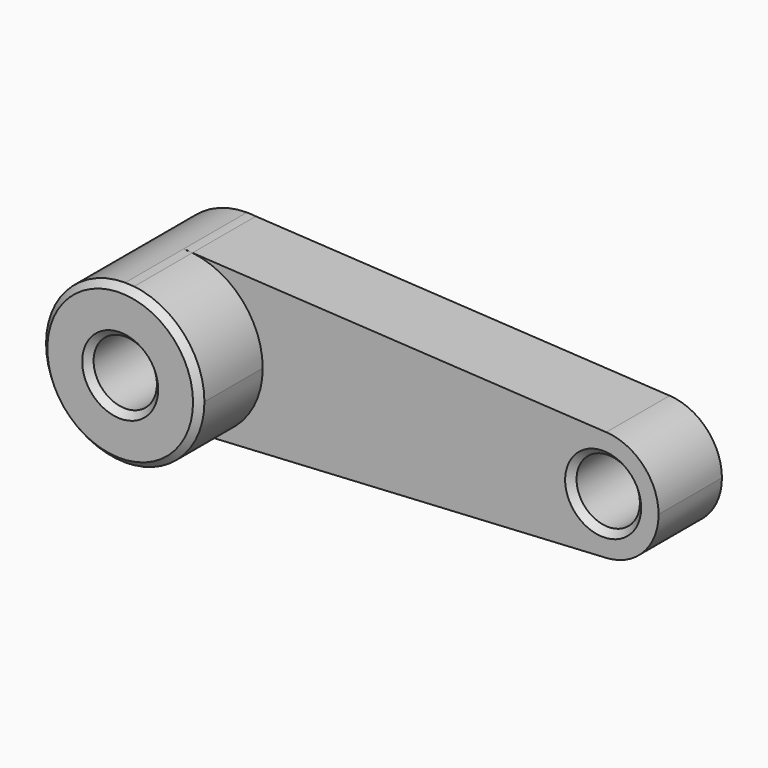
from build123d import *

# Parameters (mm, degrees)
F0_R        = 10
F1_DEPTH    = 25
F2_DEPTH    = 50
F3_T4_ANGLE = 203.6133668192
F3_T6_ANGLE = 179.9906971182


# Not quite as in the source:
# - a fillet or chamfer that OpenCascade refuses, or shapes differently, is made with other operations: its cross-section is extruded or revolved along the edge and cut away or added


with BuildPart() as f1:
    # F0 (on Front) → F1 (new body)
    with BuildSketch(Plane.XZ):
        with BuildLine():
            Line((2.8107571296, 24.8414903812), (0, 25))
            ThreePointArc((0, 25), (-25, 0), (0, -25))
            Line((0, -25), (2.8107571296, -24.8414903812))
            ThreePointArc((2.8107571296, -24.8414903812), (18.6449581421, -16.6542948179), (25, 0))
            ThreePointArc((25, 0), (18.6449581421, 16.6542948179), (2.8107571296, 24.8414903812))
        make_face()
        Circle(F0_R, mode=Mode.SUBTRACT)
        with BuildLine():
            ThreePointArc((2.8107571296, 24.8414903812), (1.4076115356, 24.9603411388), (0, 25))
            Line((0, 25), (2.8107571296, 24.8414903812))
        make_face()
        with BuildLine():
            Line((2.8107571296, -24.8414903812), (0, -25))
            ThreePointArc((0, -25), (1.4076115356, -24.9603411388), (2.8107571296, -24.8414903812))
        make_face()
        with BuildLine():
            Line((133.4853280749, 17.4722387972), (2.8107571296, 24.8414903812))
            ThreePointArc((2.8107571296, 24.8414903812), (18.6449581421, 16.6542948179), (25, 0))
            ThreePointArc((25, 0), (18.6449581421, -16.6542948179), (2.8107571296, -24.8414903812))
            Line((2.8107571296, -24.8414903812), (133.4853280749, -17.4722387972))
            ThreePointArc((133.4853280749, -17.4722387972), (115, 0), (133.4853280749, 17.4722387972))
        make_face()
        with BuildLine():
            ThreePointArc((150, 0), (145.2179644855, 12.0209558415), (133.4853280749, 17.4722387972))
            ThreePointArc((133.4853280749, 17.4722387972), (115, 0), (133.4853280749, -17.4722387972))
            ThreePointArc((133.4853280749, -17.4722387972), (145.2179644855, -12.0209558415), (150, 0))
        make_face()
        with Locations((132.5, 0)):
            Circle(F0_R, mode=Mode.SUBTRACT)
    extrude(amount=F1_DEPTH)

    # F0 (on Front) → F2 (join)
    with BuildSketch(Plane.XZ):
        with BuildLine():
            Line((2.8107571296, 24.8414903812), (0, 25))
            ThreePointArc((0, 25), (-25, 0), (0, -25))
            Line((0, -25), (2.8107571296, -24.8414903812))
            ThreePointArc((2.8107571296, -24.8414903812), (18.6449581421, -16.6542948179), (25, 0))
            ThreePointArc((25, 0), (18.6449581421, 16.6542948179), (2.8107571296, 24.8414903812))
        make_face()
        Circle(F0_R, mode=Mode.SUBTRACT)
    extrude(amount=F2_DEPTH)

    # F3: chamfer of 2 on 4 edges, made by hand

    # F3_s1 → F3_t2 (revolve, cut)
    with BuildSketch(Plane.XY):
        Polygon((12, -50), (10, -48), (10, -50), align=None)
    revolve(axis=Axis((0, -50, 0), (0, -1, 0)), mode=Mode.SUBTRACT)

    # F3_s3 → F3_t4 (revolve, cut)
    with BuildSketch(Plane(origin=(0, 0, 0), x_dir=(0, 1, 0), z_dir=(0.9788435281, 0, -0.2046102329))):
        Polygon((-48, 25), (-50, 23), (-50, 25), align=None)
    revolve(axis=Axis((0, -50, 0), (0, -1, 0)), revolution_arc=F3_T4_ANGLE, mode=Mode.SUBTRACT)

    # F3_s5 → F3_t6 (revolve, cut)
    with BuildSketch(Plane(origin=(0, 0, 0), x_dir=(0, 1, 0), z_dir=(-0.9999999967, 0, 8.1183e-05))):
        Polygon((-48, -25), (-50, -23), (-50, -25), align=None)
    revolve(axis=Axis((0, -50, 0), (0, 1, 0)), revolution_arc=F3_T6_ANGLE, mode=Mode.SUBTRACT)

    # F3_s7 → F3_t8 (revolve, cut)
    with BuildSketch(Plane.XY):
        Polygon((144.5, -25), (142.5, -23), (142.5, -25), align=None)
    revolve(axis=Axis((132.5, -25, 0), (0, -1, 0)), mode=Mode.SUBTRACT)


solid = f1.part
